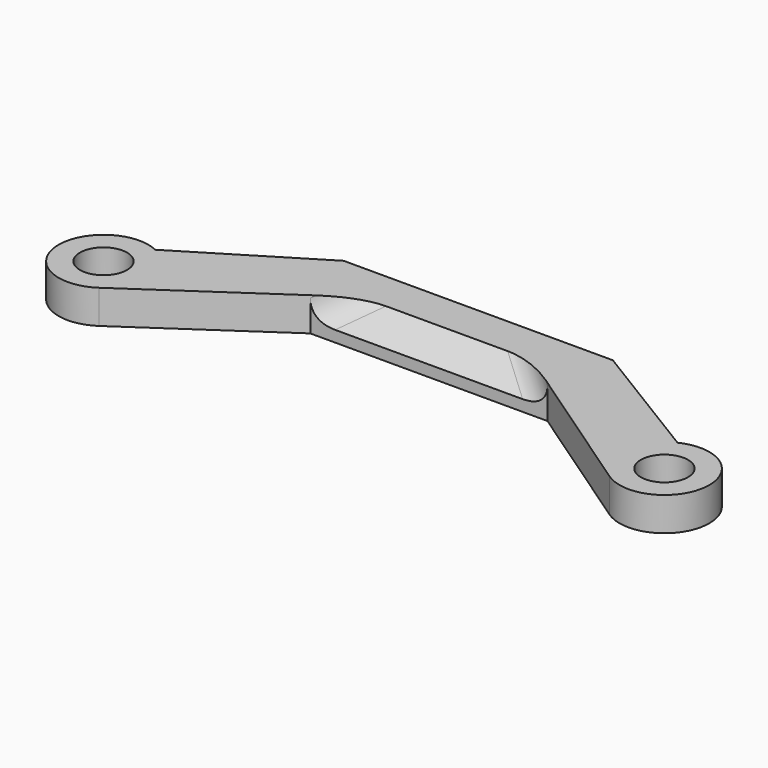
from build123d import *

# Parameters (mm, degrees)
F0_R         = 2.1
F1_DEPTH     = 3
F3_SIZE2     = 2
F3_SIZE      = 2
F4_T4_DEPTH  = 11.7592419794
F4_T10_DEPTH = 11.7592419794


# Not quite as in the source:
# - a fillet or chamfer that OpenCascade refuses, or shapes differently, is made with other operations: its cross-section is extruded or revolved along the edge and cut away or added


with BuildPart() as f1:
    # F0 (on Top) → F1 (new body)
    with BuildSketch(Plane.XY):
        with BuildLine():
            Line((0, 9), (0, 14.5))
            Line((0, 14.5), (-12, 14.5))
            Line((-12, 14.5), (-23.2738011309, 7.6083566155))
            ThreePointArc((-23.2738011309, 7.6083566155), (-28.988394733, 3.6955210129), (-22.746064478, 0.6954917669))
            Line((-22.746064478, 0.6954917669), (-10.5707757175, 9))
            Line((-10.5707757175, 9), (0, 9))
        make_face()
        with Locations((-25, 4)):
            Circle(F0_R, mode=Mode.SUBTRACT)
    extrude(amount=F1_DEPTH)

    # F2: F1 across plane


with BuildPart() as f1_1:
    add(f1.part)
    add(f1.part.mirror(Plane.YZ))

    # F3
    f3_edges = [f1_1.edges().sort_by_distance(p)[0] for p in [
        (0, 9, 3),
    ]]
    chamfer(f3_edges, length=F3_SIZE, length2=F3_SIZE2)

    # F4: fillet of radius 3 on 2 edges, made by hand


with BuildPart() as f4_tool2:
    # F4_s3 → F4_t4 (new body)
    with BuildSketch(Plane(origin=(-3.7553101229, 2.5614180039, 2.5614180039), x_dir=(0.5634838805, 0.8261270583, 0), z_dir=(0.7197293509, -0.4909122434, -0.4909122434))):
        with BuildLine():
            ThreePointArc((12.1440853808, 1.7707824696), (13.0615715756, 2.8377506524), (13.3916052457, 4.2056979457))
            Line((13.3916052457, 4.2056979457), (13.3916052457, 2.6686591321))
            Line((13.3916052457, 2.6686591321), (12.1440853808, 1.7707824696))
        make_face()
    extrude(amount=F4_T4_DEPTH)

    split(bisect_by=Plane.XY.offset(3), keep=Keep.BOTTOM)

    split(bisect_by=Plane.XZ.offset(-9), keep=Keep.BOTTOM)


with BuildPart() as f1_2:
    add(f1_1.part)

    # F4_t1: union F4_tool2
    add(f4_tool2.part)


with BuildPart() as f4_tool8:
    # F4_s9 → F4_t10 (new body)
    with BuildSketch(Plane(origin=(3.7553101229, 2.5614180039, 2.5614180039), x_dir=(0.5634838805, -0.8261270583, 0), z_dir=(-0.7197293509, -0.4909122434, -0.4909122434))):
        with BuildLine():
            ThreePointArc((-13.3916052457, 4.2056979457), (-13.0615715756, 2.8377506524), (-12.1440853808, 1.7707824696))
            Line((-12.1440853808, 1.7707824696), (-13.3916052457, 2.6686591321))
            Line((-13.3916052457, 2.6686591321), (-13.3916052457, 4.2056979457))
        make_face()
    extrude(amount=F4_T10_DEPTH)

    split(bisect_by=Plane.XY.offset(3), keep=Keep.BOTTOM)

    split(bisect_by=Plane.XZ.offset(-9), keep=Keep.BOTTOM)


with BuildPart() as f1_3:
    add(f1_2.part)

    # F4_t7: union F4_tool8
    add(f4_tool8.part)


solid = f1_3.part
